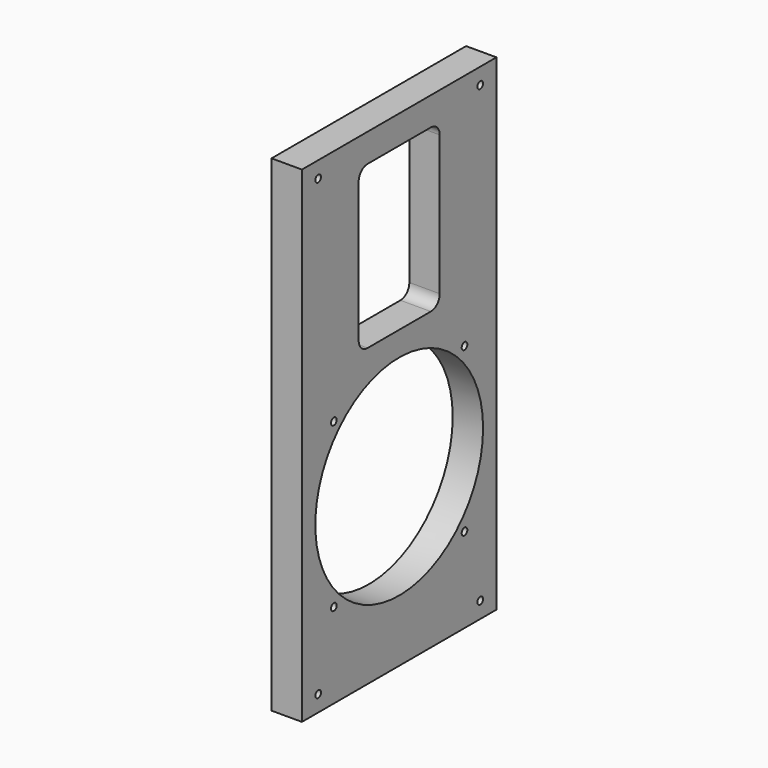
from build123d import *

# Parameters (mm, degrees)
F0_R     = 1.75
F0_R_2   = 51.75
F1_DEPTH = 15


# Not quite as in the source:
# - ends of sketch curves that miss each other by under 0.0002 mm in the source are joined


with BuildPart() as f1:
    # F0 (on Right) → F1 (new body)
    with BuildSketch(Plane.YZ):
        Polygon((-59.9995488366, -115.0645988089), (60.0004511634, -115.0645988089), (60.0004498223, 124.9354011911), (0.0004538456, 124.9354011911), (-59.9995488366, 124.9354011911), align=None)
        with Locations((-49.9999973178, -107.0645988089)):
            Circle(F0_R, mode=Mode.SUBTRACT)
        with Locations((-40.3050865276, -73.1196853366)):
            Circle(F0_R, mode=Mode.SUBTRACT)
        with Locations((0.0004511634, -32.8145988089)):
            Circle(F0_R_2, mode=Mode.SUBTRACT)
        with Locations((50.0000026822, -107.0645988089)):
            Circle(F0_R, mode=Mode.SUBTRACT)
        with Locations((40.3050865276, -73.1196853366)):
            Circle(F0_R, mode=Mode.SUBTRACT)
        with Locations((-40.3050865276, 7.4904877187)):
            Circle(F0_R, mode=Mode.SUBTRACT)
        with Locations((-49.9995488366, 116.9354011911)):
            Circle(F0_R, mode=Mode.SUBTRACT)
        with Locations((40.305537691, 7.4904877187)):
            Circle(F0_R, mode=Mode.SUBTRACT)
        with BuildLine():
            Line((-19.4991003554, 110.9354010969), (19.5008996446, 110.9354010969))
            ThreePointArc((19.5008996446, 110.9354010969), (23.3899869411, 109.3244883935), (25.0008996446, 105.4354010969))
            Line((25.0008996446, 105.4354010969), (25.0008996446, 36.4354010969))
            ThreePointArc((25.0008996446, 36.4354010969), (23.3899869411, 32.5463138004), (19.5008996446, 30.9354010969))
            Line((19.5008996446, 30.9354010969), (-19.4991003554, 30.9354010969))
            ThreePointArc((-19.4991003554, 30.9354010969), (-23.3881876519, 32.5463138004), (-24.9991003554, 36.4354010969))
            Line((-24.9991003554, 36.4354010969), (-24.9991003554, 105.4354010969))
            ThreePointArc((-24.9991003554, 105.4354010969), (-23.3881876519, 109.3244883935), (-19.4991003554, 110.9354010969))
        make_face(mode=Mode.SUBTRACT)
        with Locations((50.0004511634, 116.9354046481)):
            Circle(F0_R, mode=Mode.SUBTRACT)
    extrude(amount=-F1_DEPTH)


solid = f1.part
